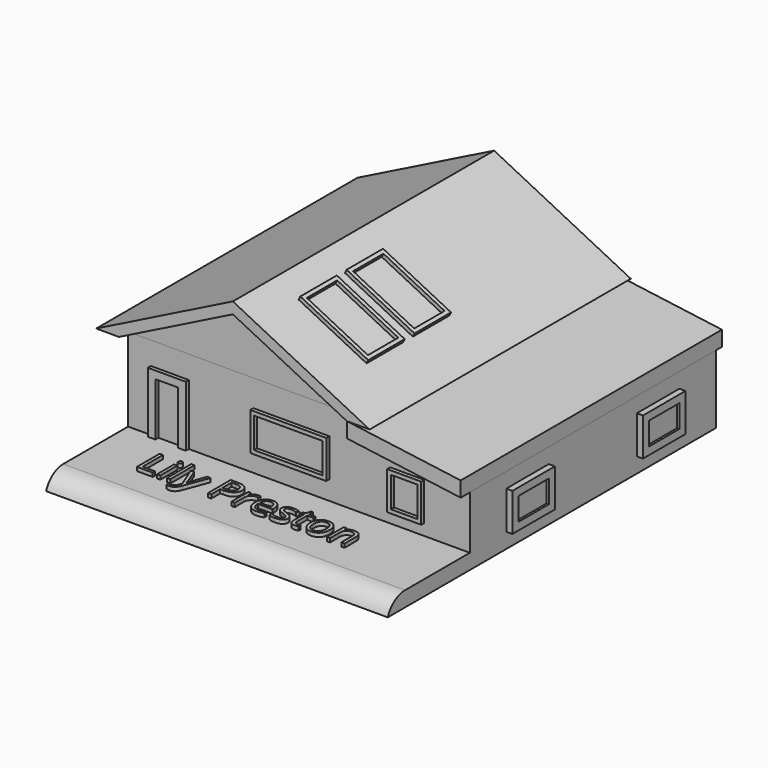
from build123d import *

# Parameters (mm, degrees)
F1_DEPTH      = 76.2
F1_DEPTH_BACK = 1016
F2_DEPTH      = 38.1
F2_DEPTH_BACK = 990.6
F0_W          = 254
F0_H          = 127
F0_W_2        = 114.3
F3_DEPTH      = 38.1
F3_DEPTH_BACK = 990.6
F0_W_3        = 228.6
F0_H_2        = 101.6
F0_W_4        = 88.9
F4_DEPTH      = 50.8
F4_DEPTH_BACK = 990.6
F0_W_5        = 76.2
F0_H_3        = 177.8
F5_DEPTH      = 38.1
F5_DEPTH_BACK = 990.6
F0_W_6        = 381
F0_H_4        = 50.8
F6_DEPTH      = 381
F6_DEPTH_BACK = 990.6
F7_T1_DEPTH   = 1502.2102448428
F8_TEXT_SIZE  = 132.8083169129
F9_DEPTH      = 12.7
F10_W         = 177.8
F10_H         = 127
F10_W_2       = 127
F10_H_2       = 76.2
F11_DEPTH     = 20.32
F12_DEPTH     = 12.7
F13_W         = 294.64
F13_H         = 167.64
F13_W_2       = 254
F13_H_2       = 127
F14_DEPTH     = 20.32
F15_DEPTH     = 12.7
F16_W         = 254
F16_H         = 152.4
F16_W_2       = 228.6
F16_H_2       = 127
F17_DEPTH     = 12.7


# Not quite as in the source:
# - a fillet or chamfer that OpenCascade refuses, or shapes differently, is made with other operations: its cross-section is extruded or revolved along the edge and cut away or added
# - Text() gives the source's letters only with a copy of the font that has no kerning and outlines rounded to 1/6400 em; it was checked with that copy


with BuildPart() as f1:
    # F0 (on Front) → F1 (new body, two sides)
    with BuildSketch(Plane.XZ) as f1_sk:
        Polygon((0, 190.5), (381, 0), (457.2, 0), (246.693881216, 105.253059392), (170.493881216, 143.353059392), (0, 228.6), (-457.2, 0), (-381, 0), align=None)
    extrude(amount=F1_DEPTH)
    extrude(f1_sk.sketch, amount=-F1_DEPTH_BACK)

    # F0 (on Front) → F2 (join, two sides)
    with BuildSketch(Plane.XZ) as f2_sk:
        Polygon((-381, 0), (0, 0), (381, 0), (0, 190.5), align=None)
    extrude(amount=F2_DEPTH)
    extrude(f2_sk.sketch, amount=-F2_DEPTH_BACK)

    # F16 (on face) → F17 (join)
    with BuildSketch(Plane(origin=(91.44, 0, 182.88), x_dir=(0.894427191, 0, -0.4472135955), z_dir=(0.4472135955, 0, 0.894427191))):
        with Locations((114.3, 174.8955229521)):
            Rectangle(F16_W, F16_H)
        with Locations((114.3, 174.8955229521)):
            Rectangle(F16_W_2, F16_H_2, mode=Mode.SUBTRACT)
        with Locations((114.3, 368.3908114433)):
            Rectangle(F16_W, F16_H)
        with Locations((114.3, 368.3908114433)):
            Rectangle(F16_W_2, F16_H_2, mode=Mode.SUBTRACT)
    extrude(amount=F17_DEPTH)


with BuildPart() as f1b:
    # F0 (on Front) → F1, piece 2 (new body, two sides)
    with BuildSketch(Plane.XZ) as f1_2_sk:
        Polygon((762, -50.8), (381, 0), (381, -50.8), (762, -101.6), align=None)
    extrude(amount=F1_DEPTH)
    extrude(f1_2_sk.sketch, amount=-F1_DEPTH_BACK)


with BuildPart() as f3:
    # F0 (on Front) → F3 (new body, two sides)
    with BuildSketch(Plane.XZ) as f3_sk:
        Polygon((381, 0), (0, 0), (-381, 0), (-381, -279.4), (-304.8, -279.4), (-304.8, -76.2), (-177.8, -76.2), (-177.8, -279.4), (381, -279.4), (381, -50.8), align=None)
        with Locations((165.1, -152.4)):
            Rectangle(F0_W, F0_H, mode=Mode.SUBTRACT)
        Polygon((762, -101.6), (381, -50.8), (381, -279.4), (762, -279.4), align=None)
        with Locations((552.45, -177.8)):
            Rectangle(F0_W_2, F0_H, mode=Mode.SUBTRACT)
    extrude(amount=F3_DEPTH)
    extrude(f3_sk.sketch, amount=-F3_DEPTH_BACK)

    # F0 (on Front) → F4 (join, two sides)
    with BuildSketch(Plane.XZ) as f4_sk:
        Polygon((-304.8, -76.2), (-304.8, -279.4), (-279.4, -279.4), (-279.4, -101.6), (-203.2, -101.6), (-203.2, -279.4), (-177.8, -279.4), (-177.8, -76.2), align=None)
        with Locations((165.1, -152.4)):
            Rectangle(F0_W, F0_H)
        with Locations((165.1, -152.4)):
            Rectangle(F0_W_3, F0_H_2, mode=Mode.SUBTRACT)
        with Locations((552.45, -177.8)):
            Rectangle(F0_W_2, F0_H)
        with Locations((552.45, -177.8)):
            Rectangle(F0_W_4, F0_H_2, mode=Mode.SUBTRACT)
    extrude(amount=F4_DEPTH)
    extrude(f4_sk.sketch, amount=-F4_DEPTH_BACK)

    # F0 (on Front) → F5 (join, two sides)
    with BuildSketch(Plane.XZ) as f5_sk:
        with Locations((-241.3, -190.5)):
            Rectangle(F0_W_5, F0_H_3)
        with Locations((165.1, -152.4)):
            Rectangle(F0_W_3, F0_H_2)
        with Locations((552.45, -177.8)):
            Rectangle(F0_W_4, F0_H_2)
    extrude(amount=F5_DEPTH)
    extrude(f5_sk.sketch, amount=-F5_DEPTH_BACK)

    # F0 (on Front) → F6 (join, two sides)
    with BuildSketch(Plane.XZ) as f6_sk:
        Polygon((-304.8, -279.4), (-381, -279.4), (-381, -330.2), (381, -330.2), (381, -279.4), (-177.8, -279.4), (-203.2, -279.4), (-279.4, -279.4), align=None)
        with Locations((571.5, -304.8)):
            Rectangle(F0_W_6, F0_H_4)
    extrude(amount=F6_DEPTH)
    extrude(f6_sk.sketch, amount=-F6_DEPTH_BACK)

    # F7: fillet of radius 76.2 on 1 edges, made by hand

    # F7_s2 → F7_t1 (cut)
    with BuildSketch(Plane.YZ.offset(-560.6051224214)):
        with BuildLine():
            ThreePointArc((-309.1579510314, -279.4), (-353.1520415437, -293.3829605333), (-381, -330.2))
            Line((-381, -330.2), (-381, -279.4))
            Line((-381, -279.4), (-309.1579510314, -279.4))
        make_face()
    extrude(amount=F7_T1_DEPTH, mode=Mode.SUBTRACT)

    # F8 (on face) → F9 (join)
    with BuildSketch(Plane.XY.offset(-279.4)):
        with Locations((-218.5121029615, -220.481403172)):
            Text('Lily Preston', F8_TEXT_SIZE, font='Open Sans', text_align=(TextAlign.LEFT, TextAlign.BOTTOM))
    extrude(amount=F9_DEPTH)

    # F10 (on face) → F11 (join)
    with BuildSketch(Plane.YZ.offset(762)):
        with Locations((203.2, -215.9)):
            Rectangle(F10_W, F10_H)
        with Locations((203.2, -215.9)):
            Rectangle(F10_W_2, F10_H_2, mode=Mode.SUBTRACT)
        with Locations((749.3, -215.9)):
            Rectangle(F10_W, F10_H)
        with Locations((749.3, -215.9)):
            Rectangle(F10_W_2, F10_H_2, mode=Mode.SUBTRACT)
    extrude(amount=F11_DEPTH)

    # F12 (add): faces of the model
    f12_faces = [f3.faces().sort_by_distance(p)[0] for p in [
        (762, 203.2, -215.9),
        (762, 749.3, -215.9),
    ]]
    extrude(f12_faces, amount=F12_DEPTH)

    # F13 (on face) → F14 (join)
    with BuildSketch(Plane(origin=(0, 990.6, 0), x_dir=(-1, 0, 0), z_dir=(0, 1, 0))):
        with Locations((-508, -191.1743494281)):
            Rectangle(F13_W, F13_H)
        with Locations((-508, -191.1743494281)):
            Rectangle(F13_W_2, F13_H_2, mode=Mode.SUBTRACT)
    extrude(amount=F14_DEPTH)

    # F15 (add): a face of the model
    f15_faces = [f3.faces().sort_by_distance(p)[0] for p in [
        (508, 990.6, -191.1743494281),
    ]]
    extrude(f15_faces, amount=F15_DEPTH)


solid = Compound([f1.part, f1b.part, f3.part])
